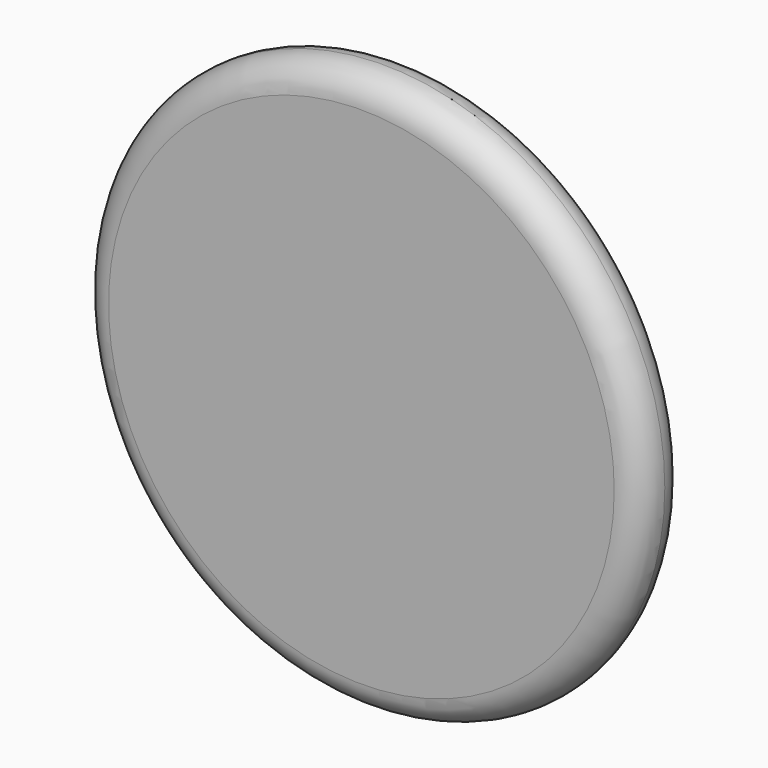
from build123d import *

# Parameters (mm, degrees)
F0_R     = 50
F1_DEPTH = 10
F2_R     = 5
F3_R     = 4.99999


# Not quite as in the source:
# - a fillet or chamfer is up to 0.001 mm smaller than in the source, because OpenCascade refuses the exact size


with BuildPart() as f1:
    # F0 (on Front) → F1 (new body)
    with BuildSketch(Plane.XZ):
        Circle(F0_R)
    extrude(amount=F1_DEPTH)

    # F2
    f2_edges = [f1.edges().sort_by_distance(p)[0] for p in [
        (-50, 0, 0),
    ]]
    fillet(f2_edges, radius=F2_R)

    # F3 (radius 5 in the source; OpenCascade refuses exactly that, so slightly less here)
    f3_edges = [f1.edges().sort_by_distance(p)[0] for p in [
        (-50, -10, 0),
        (50, -7.5, 0),
        (-50, -5, 0),
    ]]
    fillet(f3_edges, radius=F3_R)


solid = f1.part
